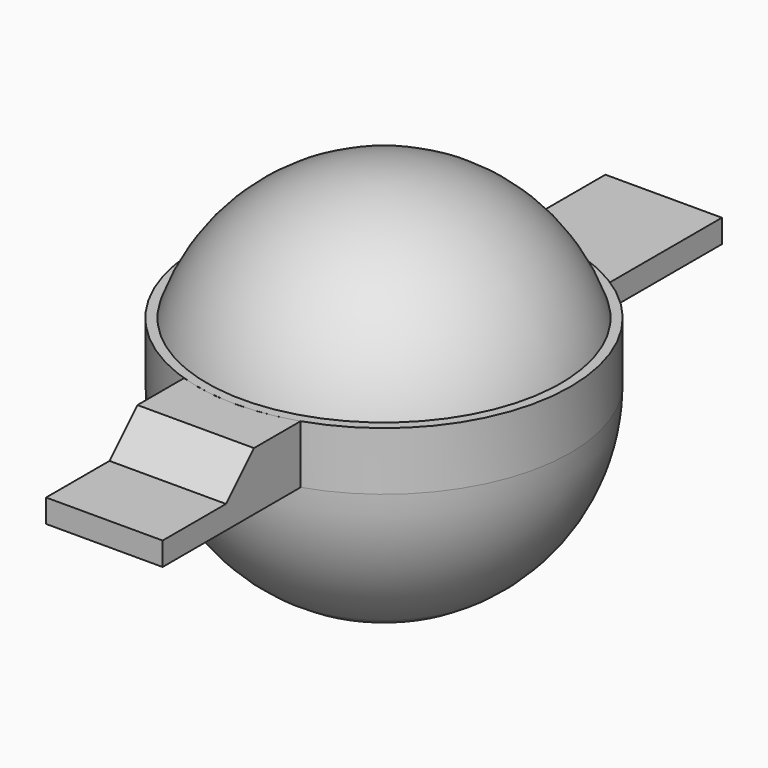
from build123d import *

# Parameters (mm, degrees)
F2_R      = 46.2010562837
F3_DEPTH  = 25
F5_R      = 29.0059042903
F6_DEPTH  = 3
F9_T      = -1.5
F10_R     = 16
F10_R_2   = 14.5
F11_DEPTH = 5
F13_DEPTH = 2
F15_DEPTH = 3
F16_SIZE  = 2.99999


# Not quite as in the source:
# - a fillet or chamfer is up to 0.001 mm smaller than in the source, because OpenCascade refuses the exact size


with BuildPart() as f1:
    # F0 (on Front) → F1 (revolve)
    with BuildSketch(Plane.XZ):
        with BuildLine():
            Line((0, 16), (0, -16))
            ThreePointArc((0, -16), (16, 0), (0, 16))
        make_face()
    revolve(axis=Axis((0, 0, 0), (0, 0, -1)))

    # F2 (on Top) → F3 (cut)
    with BuildSketch(Plane.XY):
        Circle(F2_R)
    extrude(amount=F3_DEPTH, mode=Mode.SUBTRACT)

    # F5 (on offset) → F6 (cut)
    with BuildSketch(Plane.XY.offset(-16)):
        Circle(F5_R)
    extrude(amount=F6_DEPTH, mode=Mode.SUBTRACT)


with BuildPart() as f7:
    # F0 (on Front) → F7 (revolve)
    with BuildSketch(Plane.XZ):
        with BuildLine():
            Line((0, 16), (0, -16))
            ThreePointArc((0, -16), (16, 0), (0, 16))
        make_face()
    revolve(axis=Axis((0, 0, 0), (0, 0, -1)))

    # F8: cut F1
    add(f1.part, mode=Mode.SUBTRACT)


with BuildPart() as f1_1:
    add(f1.part)

    # F9
    f9_openings = [f1_1.faces().sort_by_distance(p)[0] for p in [
        (0, 0, 0),
    ]]
    offset(amount=F9_T, openings=f9_openings)

    # F10 (on face) → F11 (join)
    with BuildSketch(Plane.XY):
        Circle(F10_R)
        Circle(F10_R_2, mode=Mode.SUBTRACT)
    extrude(amount=F11_DEPTH)


with BuildPart() as f13:
    # F12 (on Top) → F13 (new body)
    with BuildSketch(Plane.XY):
        with BuildLine():
            Line((5, -30), (5, -15.1986841536))
            ThreePointArc((5, -15.1986841536), (0, -16), (-5, -15.1986841536))
            Line((-5, -15.1986841536), (-5, -30))
            Line((-5, -30), (5, -30))
        make_face()
    extrude(amount=F13_DEPTH)

    # F14 (on face) → F15 (join, through all)
    with BuildSketch(Plane.XY.offset(5)):
        with BuildLine():
            ThreePointArc((5, -15.1986841536), (0, -16), (-5, -15.1986841536))
            Line((-5, -15.1986841536), (-5, -20.1986841536))
            Line((-5, -20.1986841536), (5, -20.1986841536))
            Line((5, -20.1986841536), (5, -15.1986841536))
        make_face()
    extrude(amount=-F15_DEPTH)

    # F16 (size 3 in the source; OpenCascade refuses exactly that, so slightly less here)
    f16_edges = [f13.edges().sort_by_distance(p)[0] for p in [
        (0, -20.198684, 2),
    ]]
    chamfer(f16_edges, length=F16_SIZE)


with BuildPart() as f13b:
    # F12 (on Top) → F13, piece 2 (new body)
    with BuildSketch(Plane.XY):
        with BuildLine():
            ThreePointArc((-5, 15.1986841536), (0, 16), (5, 15.1986841536))
            Line((5, 15.1986841536), (5, 30))
            Line((5, 30), (-5, 30))
            Line((-5, 30), (-5, 15.1986841536))
        make_face()
    extrude(amount=F13_DEPTH)


solid = Compound([f7.part, f1_1.part, f13.part, f13b.part])
